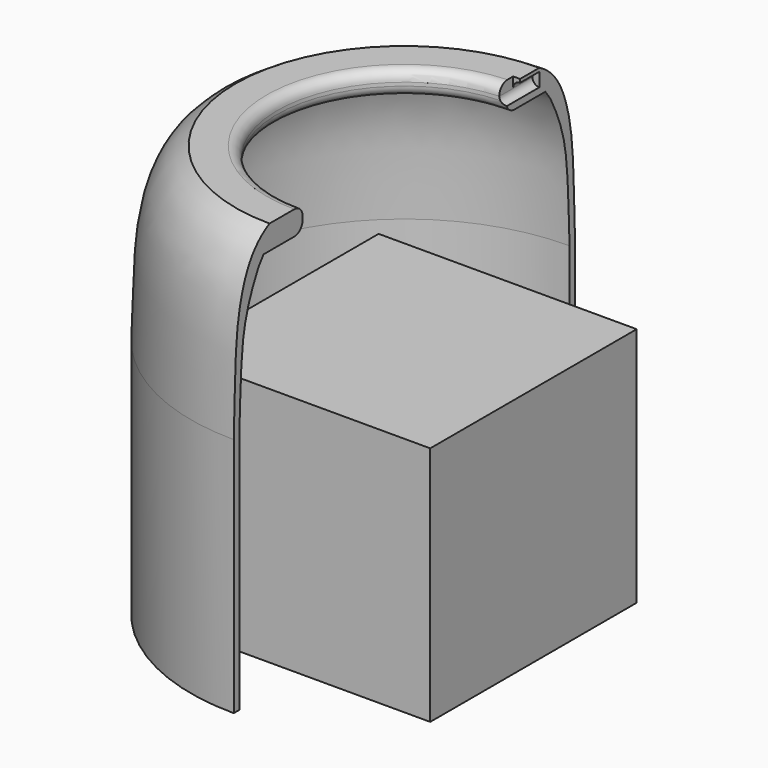
from build123d import *

# Parameters (mm, degrees)
F1_ANGLE_BACK = 90
F1_ANGLE      = 180
F3_DEPTH      = 49
F4_DEPTH      = 42
F5_W          = 75
F5_H          = 75
F6_DEPTH      = 70
F8_DEPTH      = 15
F9_R          = 1.6
F10_DEPTH     = 15
F12_R         = 4
F13_DEPTH     = 15
F14_R         = 1.6
F15_DEPTH     = 15
F17_R         = 4
F18_DEPTH     = 15


with BuildPart() as f1:
    # F0 (on Front) → F1 (revolve)
    with BuildSketch(Plane.XZ, mode=Mode.PRIVATE) as f1_sk:
        with BuildLine():
            ThreePointArc((-37, 47), (-37.8786796564, 49.1213203436), (-40, 50))
            Line((-40, 50), (-49, 50))
            add(Edge.make_bspline(
                [(-49, 50), (-50.0905438599, 49.4592544488), (-53.0493875637, 47.4989733534), (-57.4486951492, 41.931344871), (-61.5763053799, 28.0443008729), (-61.4881986154, 14.5014666819), (-62, 0)],
                knots=[0, 0, 0, 0, 0.1531073754, 0.3436852098, 0.6019385566, 1, 1, 1, 1], degree=3))
            Line((-62, 0), (-62, -70))
            Line((-62, -70), (-60, -70))
            Line((-60, -70), (-60, -0.0007486343))
            add(Edge.make_bspline(
                [(-51.1955396277, 43), (-52.5935031474, 41.0496741533), (-52.9517254174, 40.8807945198), (-59.4148587907, 27.5741318966), (-59.3836485459, 15.4725515941), (-60, -0.0007486343)],
                knots=[0, 0, 0, 0, 0.1766813791, 0.4834568095, 1, 1, 1, 1], degree=3))
            Line((-51.1955396277, 43), (-40, 43))
            ThreePointArc((-40, 43), (-37.8786796564, 43.8786796564), (-37, 46))
            Line((-37, 46), (-37, 47))
        make_face()
    revolve(f1_sk.sketch.rotate(Axis((0, 0, -69.538783133), (0, 0, 1)), -F1_ANGLE_BACK), axis=Axis((0, 0, -69.538783133), (0, 0, 1)), revolution_arc=F1_ANGLE)

    # F2 (on Front) → F3 (cut)
    with BuildSketch(Plane.XZ):
        with BuildLine():
            ThreePointArc((0, 45), (1.4142135624, 45.5857864376), (2, 47))
            ThreePointArc((2, 47), (1.4142135624, 48.4142135624), (0, 49))
            ThreePointArc((0, 49), (-1.3909130574, 48.4371363424), (-1.998931704, 47.0653608667))
            Line((-1.998931704, 47.0653608667), (-1.998931704, 46.9346391333))
            ThreePointArc((-1.998931704, 46.9346391333), (-1.3909130574, 45.5628636576), (0, 45))
        make_face()
    extrude(amount=-F3_DEPTH, mode=Mode.SUBTRACT)

    # F2 (on Front) → F4 (cut)
    with BuildSketch(Plane.XZ):
        with BuildLine():
            ThreePointArc((-1.998931704, 47.0653608667), (-1.3909130574, 48.4371363424), (0, 49))
            Line((0, 49), (0, 50.3604523001))
            Line((0, 50.3604523001), (-1.998931704, 50.3604523001))
            Line((-1.998931704, 50.3604523001), (-1.998931704, 47.0653608667))
        make_face()
    extrude(amount=-F4_DEPTH, mode=Mode.SUBTRACT)


with BuildPart() as f6:
    # F5 (on Top) → F6 (new body)
    with BuildSketch(Plane.XY):
        Rectangle(F5_W, F5_H)
    extrude(amount=-F6_DEPTH)


with BuildPart() as f8:
    # F7 (on face) → F8 (new body)
    with BuildSketch(Plane(origin=(0, 0, -70), x_dir=(1, 0, 0), z_dir=(0, 0, -1))):
        with BuildLine():
            Line((-37.5, 22.5), (-37.5, 37.5))
            Line((-37.5, 37.5), (-22.5, 37.5))
            Line((-22.5, 37.5), (-22.5, 54.5))
            ThreePointArc((-22.5, 54.5), (-41.7128787943, 41.7128787943), (-54.5, 22.5))
            Line((-54.5, 22.5), (-37.5, 22.5))
        make_face()
    extrude(amount=-F8_DEPTH)

    # F9 (on face) → F10 (cut)
    with BuildSketch(Plane.YZ.offset(-37.5)):
        with Locations((-30, -62.5)):
            Circle(F9_R)
    extrude(amount=-F10_DEPTH, mode=Mode.SUBTRACT)

    # F12 (on offset) → F13 (cut)
    with BuildSketch(Plane.YZ.offset(-60)):
        with Locations((-30, -62.5)):
            Circle(F12_R)
    extrude(amount=F13_DEPTH, mode=Mode.SUBTRACT)

    # F14 (on face) → F15 (cut)
    with BuildSketch(Plane(origin=(0, -37.5, 0), x_dir=(-1, 0, 0), z_dir=(0, 1, 0))):
        with Locations((30, -62.5)):
            Circle(F14_R)
    extrude(amount=-F15_DEPTH, mode=Mode.SUBTRACT)

    # F17 (on offset) → F18 (cut)
    with BuildSketch(Plane.XZ.offset(60)):
        with Locations((-30, -62.5)):
            Circle(F17_R)
    extrude(amount=-F18_DEPTH, mode=Mode.SUBTRACT)


solid = Compound([f1.part, f6.part, f8.part])
